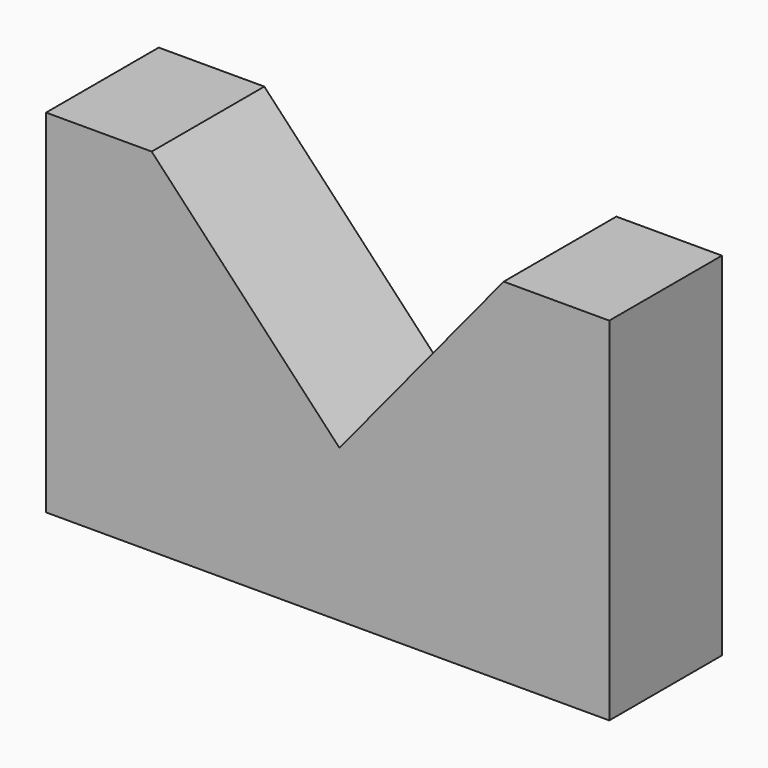
from build123d import *

# Parameters (mm, degrees)
F1_DEPTH = 25.4


# Not quite as in the source:
# - a feature names something its author has since deleted; it is built from what else it names


with BuildPart() as f1:
    # F0 (on Front) → F1 (new body)
    with BuildSketch(Plane.XZ):
        Polygon((-56.2630167723, 36.0471372604), (-75.3130167723, 36.0471372604), (-75.3130167723, -27.4528627396), (26.2869832277, -27.4528627396), (26.2869832277, 36.0471372604), (7.2369832277, 36.0471372604), (-22.3903562874, 0), align=None)
    extrude(amount=F1_DEPTH)


solid = f1.part
